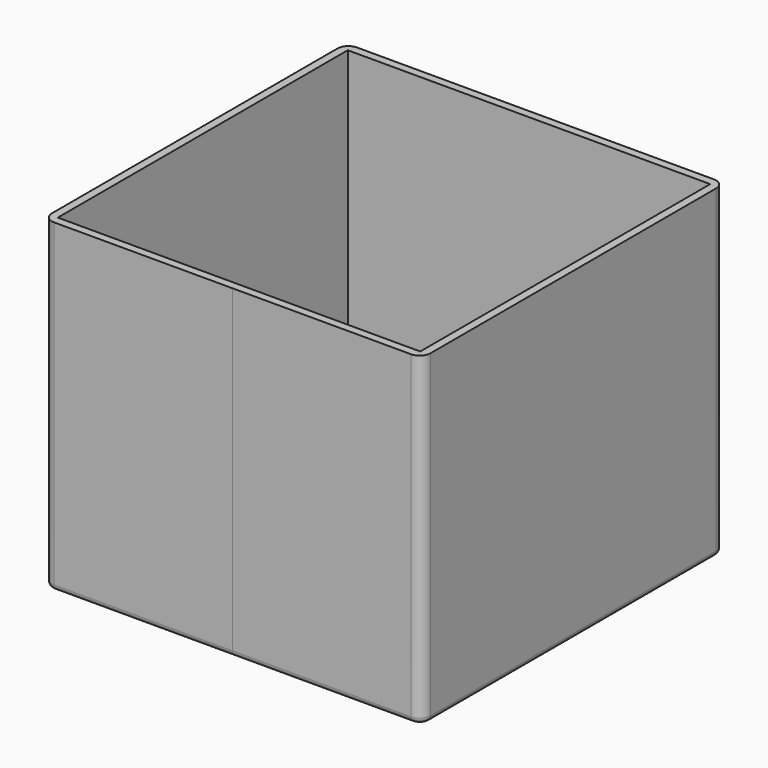
from build123d import *

# Parameters (mm, degrees)
F1_DEPTH = 152.4
F2_DEPTH = 6.35
F4_R     = 5.08
F5_R     = 2.54


# Not quite as in the source:
# - ends of sketch curves that miss each other by under 0.0002 mm in the source are joined


with BuildPart() as f1:
    # F0 (on Top) → F1 (new body)
    with BuildSketch(Plane.XY):
        Polygon((88.9, 1.431e-07), (88.9, 88.9), (0, 88.9), (0, 85.09), (85.09, 85.09), (85.09, 1.431e-07), align=None)
        Polygon((0, 85.09), (0, 88.9000001431), (-88.9, 88.9), (-88.9, 1.431e-07), (-85.09, 1.431e-07), (-85.09, 85.09), align=None)
        Polygon((-85.09, 1.431e-07), (-88.9, 1.431e-07), (-88.9, -88.9), (0, -88.9), (0, -85.09), (-85.09, -85.09), align=None)
        Polygon((88.9, -88.9), (88.9, 1.431e-07), (85.09, 1.431e-07), (85.09, -85.09), (0, -85.09), (0, -88.8999998569), align=None)
    extrude(amount=F1_DEPTH)

    # F0 (on Top) → F2 (join)
    with BuildSketch(Plane.XY):
        Polygon((85.09, -85.09), (85.09, 1.431e-07), (57.15, 1.431e-07), (44.45, 1.431e-07), (31.75, 1.431e-07), (0, 1.431e-07), (0, -31.7499998569), (10.16, -26.6699998569), (10.16, -44.4499998569), (10.16, -62.2299998569), (0, -57.1499998569), (0, -85.09), align=None)
        Polygon((0, 57.1500001431), (0, 85.09), (-85.09, 85.09), (-85.09, 1.431e-07), (-57.15, 1.431e-07), (-44.45, 1.431e-07), (-31.75, 1.431e-07), (0, 1.431e-07), (0, 31.7500001431), (-10.16, 26.6700001431), (-10.16, 44.4500001431), (-10.16, 62.2300001431), align=None)
        Polygon((44.45, 1.431e-07), (57.15, 1.431e-07), (62.23, 10.1600001431), (44.45, 10.1600001431), align=None)
        Polygon((31.75, 1.431e-07), (44.45, 1.431e-07), (44.45, 10.1600001431), (26.67, 10.1600001431), align=None)
        Polygon((0, 31.7500001431), (0, 44.4500001431), (-10.16, 44.4500001431), (-10.16, 26.6700001431), align=None)
        Polygon((0, 44.4500001431), (0, 57.1500001431), (-10.16, 62.2300001431), (-10.16, 44.4500001431), align=None)
        Polygon((85.09, 85.09), (0, 85.09), (0, 57.1500001431), (0, 44.4500001431), (0, 31.7500001431), (0, 1.431e-07), (31.75, 1.431e-07), (26.67, 10.1600001431), (44.45, 10.1600001431), (62.23, 10.1600001431), (57.15, 1.431e-07), (85.09, 1.431e-07), align=None)
        Polygon((-57.15, 1.431e-07), (-85.09, 1.431e-07), (-85.09, -85.09), (0, -85.09), (0, -57.1499998569), (0, -44.4499998569), (0, -31.7499998569), (0, 1.431e-07), (-31.75, 1.431e-07), (-26.67, -10.1599998569), (-44.45, -10.1599998569), (-62.23, -10.1599998569), align=None)
        Polygon((0, -31.7499998569), (0, -44.4499998569), (10.16, -44.4499998569), (10.16, -26.6699998569), align=None)
        Polygon((0, -44.4499998569), (0, -57.1499998569), (10.16, -62.2299998569), (10.16, -44.4499998569), align=None)
        Polygon((-31.75, 1.431e-07), (-44.45, 1.431e-07), (-44.45, -10.1599998569), (-26.67, -10.1599998569), align=None)
        Polygon((-44.45, 1.431e-07), (-57.15, 1.431e-07), (-62.23, -10.1599998569), (-44.45, -10.1599998569), align=None)
    extrude(amount=F2_DEPTH)

    # F4
    f4_edges = [f1.edges().sort_by_distance(p)[0] for p in [
        (-88.9, 88.9, 76.2),
        (88.9, 88.9, 76.2),
        (88.9, -88.9, 76.2),
        (-88.9, -88.9, 76.2),
    ]]
    fillet(f4_edges, radius=F4_R)

    # F5
    f5_edges = [f1.edges().sort_by_distance(p)[0] for p in [
        (41.91, 88.9, 0),
        (87.412102, 87.412102, 0),
        (-41.91, 88.9, 0),
        (88.9, 0, 0),
        (-87.412102, 87.412102, 0),
        (87.412102, -87.412102, 0),
        (-88.9, 0, 0),
        (41.91, -88.9, 0),
        (-87.412102, -87.412102, 0),
        (-41.91, -88.9, 0),
    ]]
    fillet(f5_edges, radius=F5_R)


solid = f1.part
